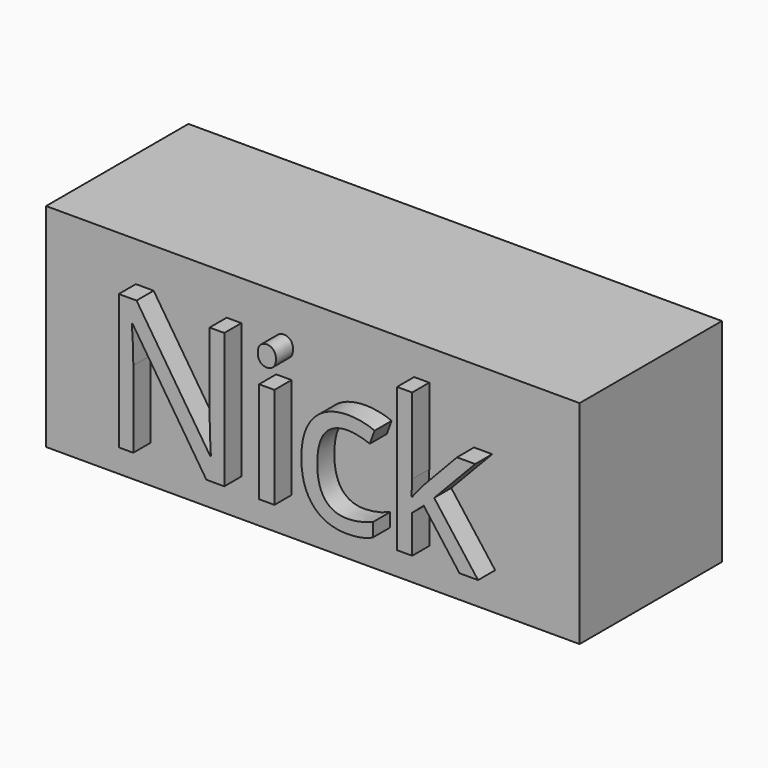
from build123d import *

# Parameters (mm, degrees)
F0_W         = 76.1828105897
F0_H         = 30.2911140025
F1_DEPTH     = 25.4
F2_TEXT_SIZE = 27.0122739797
F3_DEPTH     = 3.048


# Not quite as in the source:
# - Text() gives the source's letters only with a copy of the font that has no kerning and outlines rounded to 1/6400 em; it was checked with that copy


with BuildPart() as f1:
    # F0 (on Front) → F1 (new body)
    with BuildSketch(Plane.XZ):
        with Locations((10.715582408, 39.3451806158)):
            Rectangle(F0_W, F0_H)
    extrude(amount=F1_DEPTH)

    # F2 (on face) → F3 (join)
    with BuildSketch(Plane.XZ.offset(25.4)):
        with Locations((-17.204226926, 29.5607391745)):
            Text('Nick', F2_TEXT_SIZE, font='Open Sans', text_align=(TextAlign.LEFT, TextAlign.BOTTOM))
    extrude(amount=F3_DEPTH)


solid = f1.part
